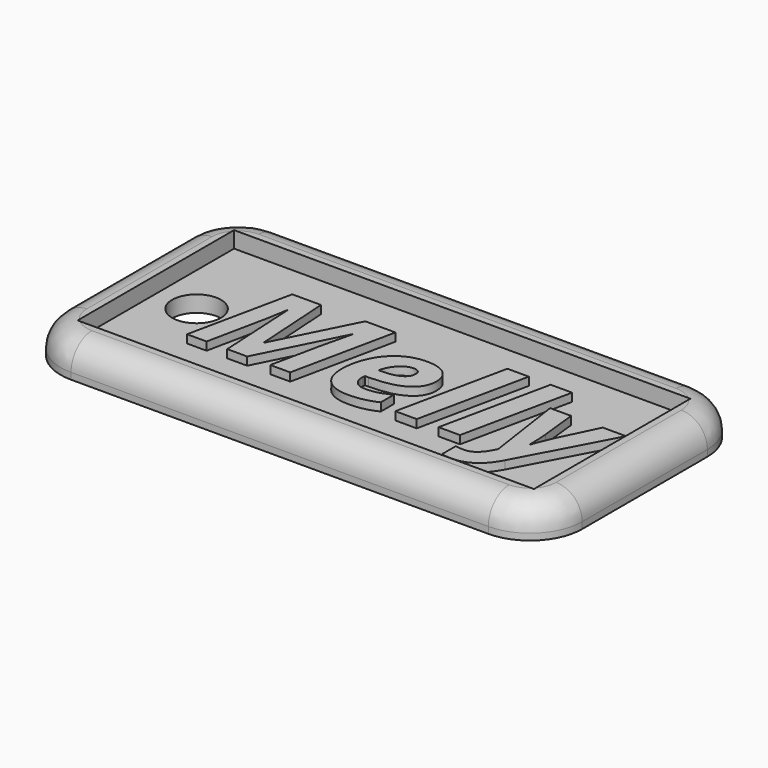
from build123d import *

# Parameters (mm, degrees)
F0_W         = 44.45
F0_H         = 19.05
F0_R         = 2.38125
F1_DEPTH     = 1.5875
F0_W_2       = 50.8
F0_H_2       = 25.4
F2_DEPTH     = 3.175
F3_R         = 5.08
F4_T1_DEPTH  = 40.64
F4_T3_DEPTH  = 15.24
F4_T6_ANGLE  = 90
F4_T8_ANGLE  = 90
F4_T10_ANGLE = 90
F4_T12_ANGLE = 90
F5_TEXT_SIZE = 14.194442072
F6_DEPTH     = 0.79375


# Not quite as in the source:
# - a fillet or chamfer that OpenCascade refuses, or shapes differently, is made with other operations: its cross-section is extruded or revolved along the edge and cut away or added
# - Text() gives the source's letters only with a copy of the font that has no kerning and outlines rounded to 1/6400 em; it was checked with that copy


with BuildPart() as f1:
    # F0 (on Top) → F1 (new body)
    with BuildSketch(Plane.XY):
        with Locations((25.4, 12.7)):
            Rectangle(F0_W, F0_H)
        with Locations((7.14375, 12.7)):
            Circle(F0_R, mode=Mode.SUBTRACT)
    extrude(amount=F1_DEPTH)

    # F0 (on Top) → F2 (join)
    with BuildSketch(Plane.XY):
        with Locations((25.4, 12.7)):
            Rectangle(F0_W_2, F0_H_2)
        with Locations((25.4, 12.7)):
            Rectangle(F0_W, F0_H, mode=Mode.SUBTRACT)
    extrude(amount=F2_DEPTH)

    # F3
    f3_edges = [f1.edges().sort_by_distance(p)[0] for p in [
        (0, 0, 1.5875),
        (50.8, 0, 1.5875),
        (50.8, 25.4, 1.5875),
        (0, 25.4, 1.5875),
    ]]
    fillet(f3_edges, radius=F3_R)

    # F4: fillet of radius 2.54 on 8 edges, made by hand

    # F4_s2 → F4_t1 (cut)
    with BuildSketch(Plane.YZ.offset(5.08)):
        with BuildLine():
            ThreePointArc((0, 0.635), (0.7439487758, 2.4310512242), (2.54, 3.175))
            Line((2.54, 3.175), (0, 3.175))
            Line((0, 3.175), (0, 0.635))
        make_face()
        with BuildLine():
            ThreePointArc((25.4, 0.635), (24.6560512242, 2.4310512242), (22.86, 3.175))
            Line((22.86, 3.175), (25.4, 3.175))
            Line((25.4, 3.175), (25.4, 0.635))
        make_face()
    extrude(amount=F4_T1_DEPTH, mode=Mode.SUBTRACT)

    # F4_s4 → F4_t3 (cut)
    with BuildSketch(Plane.XZ.offset(-20.32)):
        with BuildLine():
            ThreePointArc((0, 0.635), (0.7439487758, 2.4310512242), (2.54, 3.175))
            Line((2.54, 3.175), (0, 3.175))
            Line((0, 3.175), (0, 0.635))
        make_face()
        with BuildLine():
            ThreePointArc((50.8, 0.635), (50.0560512242, 2.4310512242), (48.26, 3.175))
            Line((48.26, 3.175), (50.8, 3.175))
            Line((50.8, 3.175), (50.8, 0.635))
        make_face()
    extrude(amount=F4_T3_DEPTH, mode=Mode.SUBTRACT)

    # F4_s5 → F4_t6 (revolve, cut)
    with BuildSketch(Plane.XZ.offset(-20.32)):
        with BuildLine():
            ThreePointArc((0, 0.635), (0.7439487758, 2.4310512242), (2.54, 3.175))
            Line((2.54, 3.175), (0, 3.175))
            Line((0, 3.175), (0, 0.635))
        make_face()
    revolve(axis=Axis((5.08, 20.32, 3.175), (0, 0, -1)), revolution_arc=F4_T6_ANGLE, mode=Mode.SUBTRACT)

    # F4_s7 → F4_t8 (revolve, cut)
    with BuildSketch(Plane.XZ.offset(-5.08)):
        with BuildLine():
            ThreePointArc((0, 0.635), (0.7439487758, 2.4310512242), (2.54, 3.175))
            Line((2.54, 3.175), (0, 3.175))
            Line((0, 3.175), (0, 0.635))
        make_face()
    revolve(axis=Axis((5.08, 5.08, 3.175), (0, 0, 1)), revolution_arc=F4_T8_ANGLE, mode=Mode.SUBTRACT)

    # F4_s9 → F4_t10 (revolve, cut)
    with BuildSketch(Plane.XZ.offset(-20.32)):
        with BuildLine():
            ThreePointArc((50.8, 0.635), (50.0560512242, 2.4310512242), (48.26, 3.175))
            Line((48.26, 3.175), (50.8, 3.175))
            Line((50.8, 3.175), (50.8, 0.635))
        make_face()
    revolve(axis=Axis((45.72, 20.32, 3.175), (0, 0, 1)), revolution_arc=F4_T10_ANGLE, mode=Mode.SUBTRACT)

    # F4_s11 → F4_t12 (revolve, cut)
    with BuildSketch(Plane.YZ.offset(45.72)):
        with BuildLine():
            ThreePointArc((0, 0.635), (0.7439487758, 2.4310512242), (2.54, 3.175))
            Line((2.54, 3.175), (0, 3.175))
            Line((0, 3.175), (0, 0.635))
        make_face()
    revolve(axis=Axis((45.72, 5.08, 3.175), (0, 0, 1)), revolution_arc=F4_T12_ANGLE, mode=Mode.SUBTRACT)

    # F5 (on face) → F6 (join)
    with BuildSketch(Plane.XY.offset(1.5875)):
        with Locations((9.7768509441, 7.7871199631)):
            Text('Melly', F5_TEXT_SIZE, font='Open Sans', font_style=FontStyle.BOLDITALIC, text_align=(TextAlign.LEFT, TextAlign.BOTTOM))
    extrude(amount=F6_DEPTH)


solid = f1.part
